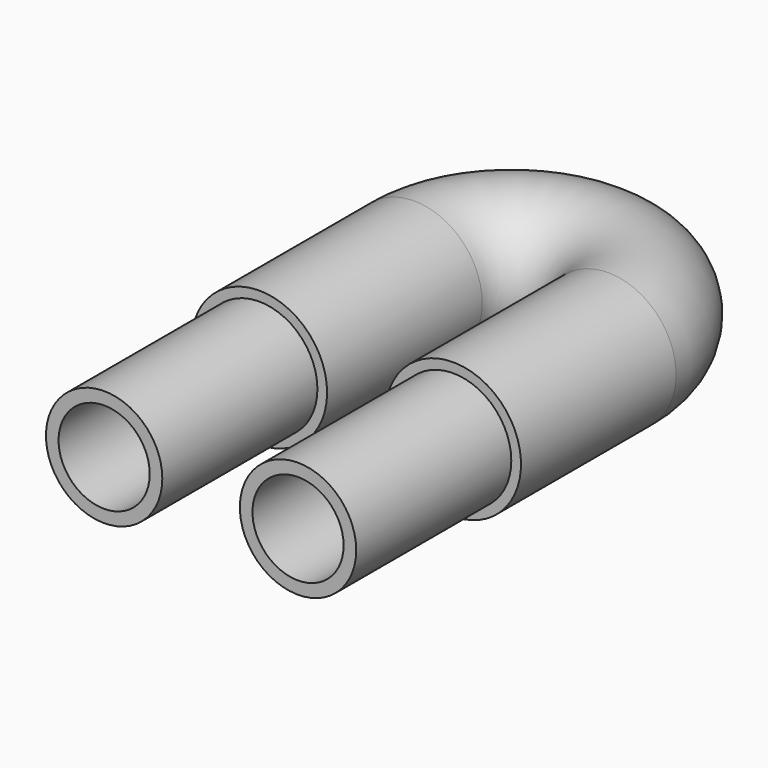
from build123d import *
from build123d import SkipClean  # not in build123d's __all__

# Parameters (mm, degrees)
F0_R     = 8.89
F0_R_2   = 5.969
F3_R     = 7.62
F3_R_2   = 5.969
F4_R     = 7.62
F4_R_2   = 5.969
F5_DEPTH = 25.4


with BuildPart() as f2:
    # F2: sweep along a path in F1
    with BuildLine(Plane.XY) as f2_path:
        Line((0, 0), (0, 25.4))
        ThreePointArc((0, 25.4), (12.7, 38.1), (25.4, 25.4))
        Line((25.4, 25.4), (25.4, 0))
    # F0 (on Front) → F2 (sweep)
    with BuildSketch(Plane.XZ):
        Circle(F0_R)
        Circle(F0_R_2, mode=Mode.SUBTRACT)
    sweep(path=f2_path.line)

    # F3 (on face) + F4 (on face) → F5 (join)
    with BuildSketch(Plane.XZ):
        Circle(F3_R)
        Circle(F3_R_2, mode=Mode.SUBTRACT)
    with BuildSketch(Plane.XZ):
        with Locations((25.4, 0)):
            Circle(F4_R)
        with Locations((25.4, 0)):
            Circle(F4_R_2, mode=Mode.SUBTRACT)
    with SkipClean():  # cleaning this boolean's faces spoils the solid; the shape is the same uncleaned
        extrude(amount=F5_DEPTH)


solid = f2.part
